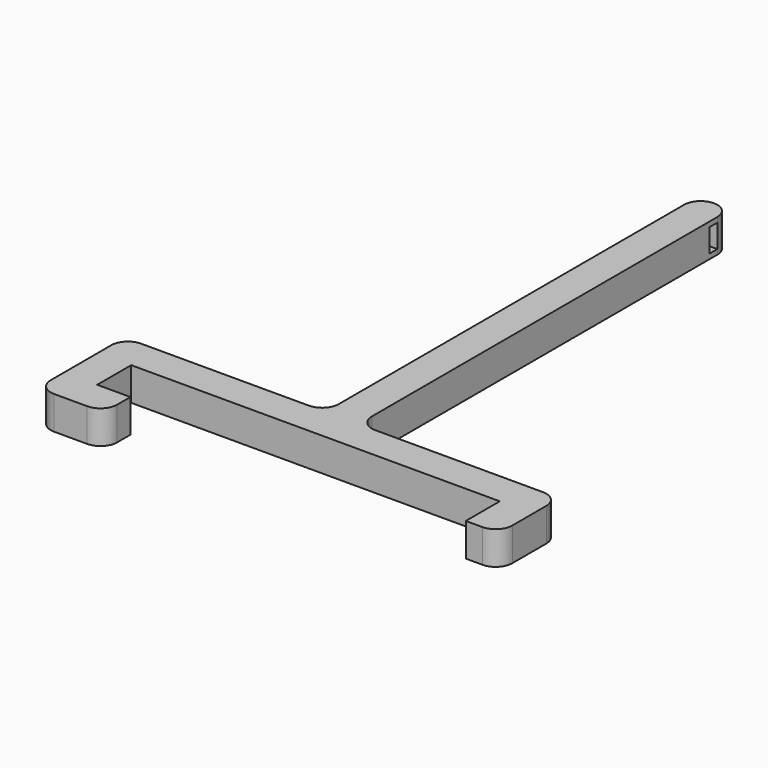
from build123d import *

# Parameters (mm, degrees)
F0_W     = 5
F0_H     = 6.4
F1_DEPTH = 5
F2_W     = 5
F2_H     = 5
F3_DEPTH = 70
F4_W     = 1.5
F4_H     = 3.5
F5_DEPTH = 5
F6_R     = 2.49999


# Not quite as in the source:
# - a fillet or chamfer is up to 0.001 mm smaller than in the source, because OpenCascade refuses the exact size


with BuildPart() as f1:
    # F0 (on Top) → F1 (new body)
    with BuildSketch(Plane.XY):
        with Locations((30.25, 0)):
            Rectangle(F0_W, F0_H)
        Polygon((-27.75, 3.2), (27.75, 3.2), (32.75, 3.2), (32.75, 8.2), (-27.75, 8.2), align=None)
        Polygon((-27.75, -3.2), (-27.75, 3.2), (-27.75, 8.2), (-32.75, 8.2), (-32.75, -3.2), align=None)
        Polygon((-22.75, -3.2), (-27.75, -3.2), (-32.75, -3.2), (-32.75, -8.2), (-22.75, -8.2), align=None)
    extrude(amount=F1_DEPTH)

    # F2 (on face) → F3 (join)
    with BuildSketch(Plane(origin=(0, 8.2, 0), x_dir=(-1, 0, 0), z_dir=(0, 1, 0))):
        with Locations((0, 2.5)):
            Rectangle(F2_W, F2_H)
    extrude(amount=F3_DEPTH)

    # F4 (on face) → F5 (cut, through all)
    with BuildSketch(Plane.YZ.offset(2.5)):
        with Locations((74.95, 2.5)):
            Rectangle(F4_W, F4_H)
    extrude(amount=-F5_DEPTH, mode=Mode.SUBTRACT)

    # F6 (radius 2.5 in the source; OpenCascade refuses exactly that, so slightly less here)
    f6_edges = [f1.edges().sort_by_distance(p)[0] for p in [
        (32.75, 8.2, 2.5),
        (2.5, 8.2, 2.5),
        (-2.5, 8.2, 2.5),
        (-32.75, 8.2, 2.5),
        (32.75, -3.2, 2.5),
        (-32.75, -8.2, 2.5),
        (-22.75, -8.2, 2.5),
        (-2.5, 78.2, 2.5),
        (2.5, 78.2, 2.5),
    ]]
    fillet(f6_edges, radius=F6_R)


solid = f1.part
